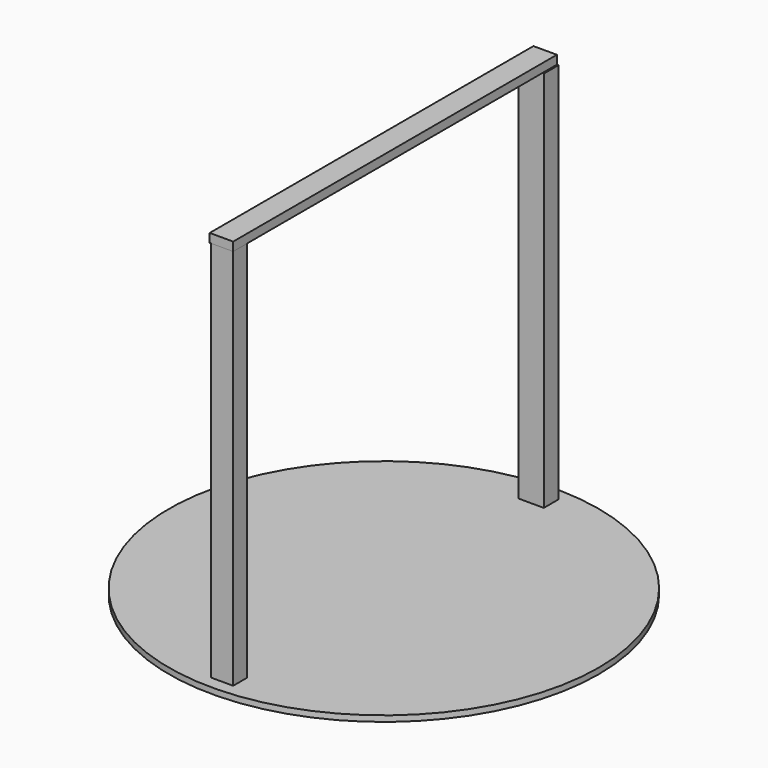
from build123d import *

# Parameters (mm, degrees)
F1_W     = 3.897249233
F1_H     = 2.9796436429
F2_DEPTH = 66.802
F1_W_2   = 4.4288989156
F1_H_2   = 3.24241817
F3_W     = 4.099171143
F3_H     = 70.7048140466
F4_DEPTH = 1.524
F0_R     = 37.5629925572
F5_DEPTH = 1.016


# Not quite as in the source:
# - the program builds the solid bodies; features that only make, move or delete a surface that nothing else refers to are left out


with BuildPart() as f2:
    # F1 (on face) → F2 (new body)
    with BuildSketch(Plane.XY):
        with Locations((0, -33.859655261)):
            Rectangle(F1_W, F1_H)
    extrude(amount=F2_DEPTH)


with BuildPart() as f2b:
    # F1 (on face) → F2, piece 2 (new body)
    with BuildSketch(Plane.XY):
        with Locations((0, 33.7925106287)):
            Rectangle(F1_W_2, F1_H_2)
    extrude(amount=F2_DEPTH)


with BuildPart() as f4:
    # F3 (on face) → F4 (new body)
    with BuildSketch(Plane.XY.offset(66.802)):
        with Locations((-0.100960955, 0.0029299408)):
            Rectangle(F3_W, F3_H)
    extrude(amount=F4_DEPTH)


with BuildPart() as f5:
    # F0 (on Top) → F5 (new body)
    with BuildSketch(Plane.XY):
        Circle(F0_R)
    extrude(amount=-F5_DEPTH)


solid = Compound([f2.part, f2b.part, f4.part, f5.part])
